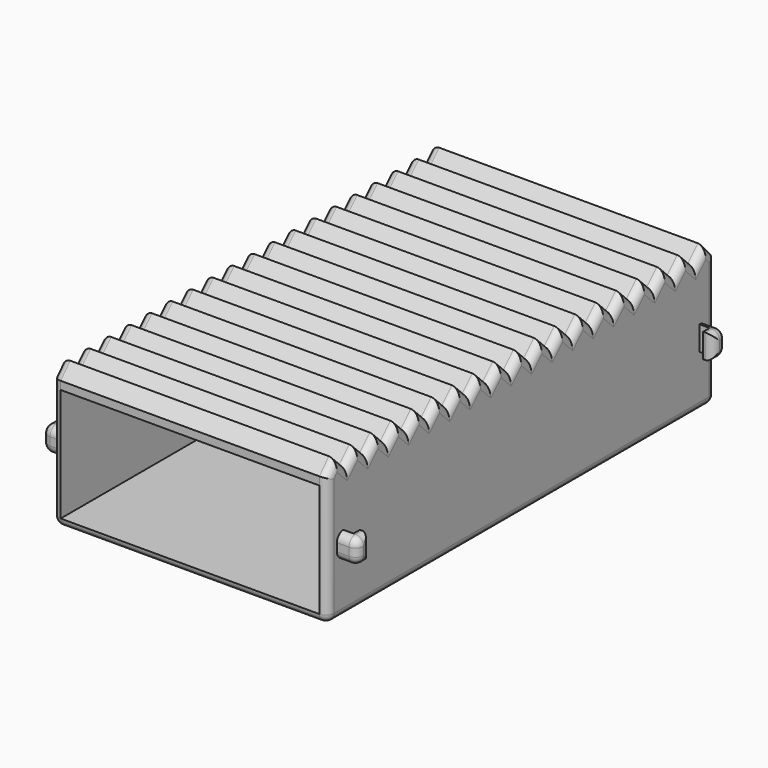
from build123d import *

# Parameters (mm, degrees)
F0_W     = 34
F0_H     = 16
F0_W_2   = 32
F0_H_2   = 14
F1_DEPTH = 30
F3_DEPTH = 34
F4_R     = 0.99999
F7_DEPTH = 1.5
F8_R     = 0.99999


# Not quite as in the source:
# - a fillet or chamfer is up to 0.001 mm smaller than in the source, because OpenCascade refuses the exact size


with BuildPart() as f1:
    # F0 (on Front) → F1 (new body, symmetric)
    with BuildSketch(Plane.XZ):
        with Locations((0, 8)):
            Rectangle(F0_W, F0_H)
        with Locations((0, 8)):
            Rectangle(F0_W_2, F0_H_2, mode=Mode.SUBTRACT)
    extrude(amount=F1_DEPTH, both=True)

    # F2 (on face) → F3 (join)
    with BuildSketch(Plane.YZ.offset(17)):
        Polygon((-28.529796507, 17.5949886948), (-30, 16), (30, 16), (28.529796507, 17.5949886948), (26.9448078121, 16.01), (25.3598191173, 17.5949886948), (23.7748304225, 16.01), (22.1898417276, 17.5949886948), (20.6048530328, 16.01), (19.019864338, 17.5949886948), (17.4348756431, 16.01), (15.8498869483, 17.5949886948), (14.2648982535, 16.01), (12.6799095586, 17.5949886948), (11.0949208638, 16.01), (9.509932169, 17.5949886948), (7.9249434742, 16.01), (6.3399547793, 17.5949886948), (4.7549660845, 16.01), (3.1699773897, 17.5949886948), (1.5849886948, 16.01), (0, 17.5949886948), (-1.5849886948, 16.01), (-3.1699773897, 17.5949886948), (-4.7549660845, 16.01), (-6.3399547793, 17.5949886948), (-7.9249434742, 16.01), (-9.509932169, 17.5949886948), (-11.0949208638, 16.01), (-12.6799095586, 17.5949886948), (-14.2648982535, 16.01), (-15.8498869483, 17.5949886948), (-17.4348756431, 16.01), (-19.019864338, 17.5949886948), (-20.6048530328, 16.01), (-22.1898417276, 17.5949886948), (-23.7748304225, 16.01), (-25.3598191173, 17.5949886948), (-26.9448078121, 16.01), align=None)
    extrude(amount=-F3_DEPTH)

    # F4 (radius 1 in the source; OpenCascade refuses exactly that, so slightly less here)
    f4_edges = [f1.edges().sort_by_distance(p)[0] for p in [
        (17, 0, 0),
        (17, 30, 8),
        (17, 29.264898, 16.797494),
        (17, 27.737302, 16.802494),
        (17, 26.152313, 16.802494),
        (17, 24.567325, 16.802494),
        (17, 22.982336, 16.802494),
        (17, 21.397347, 16.802494),
        (17, 19.812359, 16.802494),
        (17, 18.22737, 16.802494),
        (17, 16.642381, 16.802494),
        (17, 15.057393, 16.802494),
        (17, 13.472404, 16.802494),
        (17, 11.887415, 16.802494),
        (17, 10.302427, 16.802494),
        (17, 8.717438, 16.802494),
        (17, 7.132449, 16.802494),
        (17, 5.54746, 16.802494),
        (17, 3.962472, 16.802494),
        (17, 2.377483, 16.802494),
        (17, 0.792494, 16.802494),
        (17, -0.792494, 16.802494),
        (17, -2.377483, 16.802494),
        (17, -3.962472, 16.802494),
        (17, -5.54746, 16.802494),
        (17, -7.132449, 16.802494),
        (17, -8.717438, 16.802494),
        (17, -10.302427, 16.802494),
        (17, -11.887415, 16.802494),
        (17, -13.472404, 16.802494),
        (17, -15.057393, 16.802494),
        (17, -16.642381, 16.802494),
        (17, -18.22737, 16.802494),
        (17, -19.812359, 16.802494),
        (17, -21.397347, 16.802494),
        (17, -22.982336, 16.802494),
        (17, -24.567325, 16.802494),
        (17, -26.152313, 16.802494),
        (17, -27.737302, 16.802494),
        (17, -29.264898, 16.797494),
        (17, -30, 8),
        (-17, 0, 0),
        (0, 30, 0),
        (0, -30, 0),
        (-17, 30, 8),
        (-17, -30, 8),
        (-17, -29.264898, 16.797494),
        (-17, -27.737302, 16.802494),
        (-17, -26.152313, 16.802494),
        (-17, -24.567325, 16.802494),
        (-17, -22.982336, 16.802494),
        (-17, -21.397347, 16.802494),
        (-17, -19.812359, 16.802494),
        (-17, -18.22737, 16.802494),
        (-17, -16.642381, 16.802494),
        (-17, -15.057393, 16.802494),
        (-17, -13.472404, 16.802494),
        (-17, -11.887415, 16.802494),
        (-17, -10.302427, 16.802494),
        (-17, -8.717438, 16.802494),
        (-17, -7.132449, 16.802494),
        (-17, -5.54746, 16.802494),
        (-17, -3.962472, 16.802494),
        (-17, -2.377483, 16.802494),
        (-17, -0.792494, 16.802494),
        (-17, 0.792494, 16.802494),
        (-17, 2.377483, 16.802494),
        (-17, 3.962472, 16.802494),
        (-17, 5.54746, 16.802494),
        (-17, 7.132449, 16.802494),
        (-17, 8.717438, 16.802494),
        (-17, 10.302427, 16.802494),
        (-17, 11.887415, 16.802494),
        (-17, 13.472404, 16.802494),
        (-17, 15.057393, 16.802494),
        (-17, 16.642381, 16.802494),
        (-17, 18.22737, 16.802494),
        (-17, 19.812359, 16.802494),
        (-17, 21.397347, 16.802494),
        (-17, 22.982336, 16.802494),
        (-17, 24.567325, 16.802494),
        (-17, 26.152313, 16.802494),
        (-17, 27.737302, 16.802494),
        (-17, 29.264898, 16.797494),
    ]]
    fillet(f4_edges, radius=F4_R)

    # F6 (on offset) → F7 (join, symmetric)
    with BuildSketch(Plane.XY.offset(8)):
        Polygon((17, -27.529796507), (17, -28.529796507), (19.5, -28.529796507), (19.5, -26.529796507), (18.25, -26.529796507), (18.25, -27.529796507), align=None)
        Polygon((-19.5, -28.529796507), (-17, -28.529796507), (-17, -27.529796507), (-18.25, -27.529796507), (-18.25, -26.529796507), (-19.5, -26.529796507), align=None)
        Polygon((-17, 28.529796507), (-19.5, 28.529796507), (-19.5, 26.529796507), (-18.25, 26.529796507), (-18.25, 27.529796507), (-17, 27.529796507), align=None)
        Polygon((18.25, 27.529796507), (18.25, 26.529796507), (19.5, 26.529796507), (19.5, 28.529796507), (17, 28.529796507), (17, 27.529796507), align=None)
    extrude(amount=F7_DEPTH, both=True)

    # F8 (radius 1 in the source; OpenCascade refuses exactly that, so slightly less here)
    f8_edges = [f1.edges().sort_by_distance(p)[0] for p in [
        (-19.5, 28.529797, 8),
        (-18.25, 28.529797, 9.5),
        (-18.25, 28.529797, 6.5),
        (-19.5, 27.529797, 6.5),
        (-19.5, 26.529797, 8),
        (-19.5, 27.529797, 9.5),
        (18.25, 28.529797, 9.5),
        (18.25, 28.529797, 6.5),
        (19.5, 26.529797, 8),
        (19.5, 27.529797, 6.5),
        (19.5, 28.529797, 8),
        (19.5, 27.529797, 9.5),
        (18.25, -28.529797, 9.5),
        (18.25, -28.529797, 6.5),
        (19.5, -28.529797, 8),
        (19.5, -27.529797, 6.5),
        (19.5, -26.529797, 8),
        (19.5, -27.529797, 9.5),
        (-19.5, -27.529797, 6.5),
        (-19.5, -28.529797, 8),
        (-19.5, -27.529797, 9.5),
        (-19.5, -26.529797, 8),
        (-18.25, -28.529797, 9.5),
        (-18.25, -28.529797, 6.5),
    ]]
    fillet(f8_edges, radius=F8_R)


solid = f1.part
